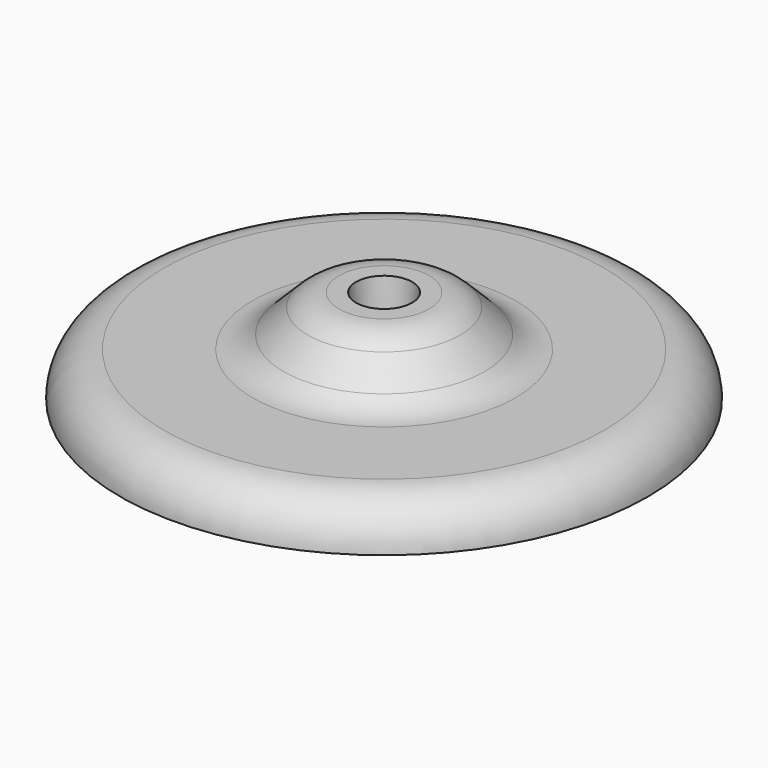
from build123d import *

# Parameters (mm, degrees)
F2_R = 4.99999


# Not quite as in the source:
# - a fillet or chamfer is up to 0.001 mm smaller than in the source, because OpenCascade refuses the exact size


with BuildPart() as f1:
    # F0 (on Front) → F1 (revolve)
    with BuildSketch(Plane.XZ):
        Polygon((30, 5), (12.8825559993, 5), (7.1957559993, 10.6868), (3.1957559993, 10.6868), (2.6416, 2.762), (2.6416, 2), (0, 2), (0, 0), (30, 0), align=None)
    revolve(axis=Axis((0, 0, -11.1281685531), (0, 0, -1)))

    # F2 (radius 5 in the source; OpenCascade refuses exactly that, so slightly less here)
    f2_edges = [f1.edges().sort_by_distance(p)[0] for p in [
        (-12.882556, 0, 5),
        (-30, 0, 5),
        (-7.195756, 0, 10.6868),
    ]]
    fillet(f2_edges, radius=F2_R)


solid = f1.part
